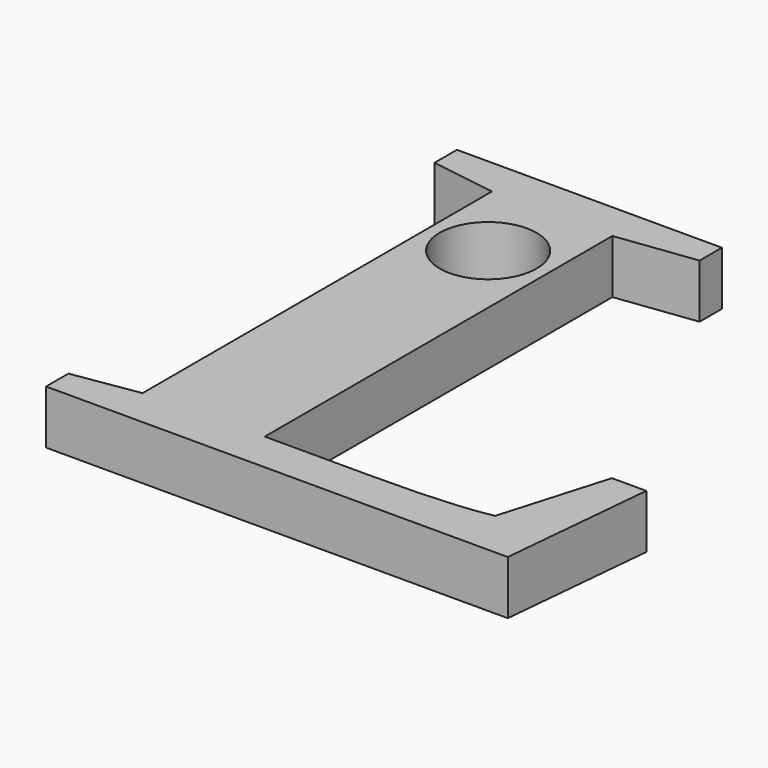
from build123d import *

# Parameters (mm, degrees)
F0_TEXT_SIZE = 72.7272727273
F1_DEPTH     = 5
F3_D         = 9


# Not quite as in the source:
# - Text() gives the source's letters only with a copy of the font that has no kerning and outlines rounded to 1/6400 em; it was checked with that copy


with BuildPart() as f1:
    # F0 (on Top) → F1 (new body)
    with BuildSketch(Plane.XY):
        with Locations((-41.6577126533, -22.5778426675)):
            Text('L', F0_TEXT_SIZE, font='Tinos', font_style=FontStyle.BOLD, text_align=(TextAlign.LEFT, TextAlign.BOTTOM))
    extrude(amount=F1_DEPTH)

    # F3 (through all)
    with Locations(Plane.XY.offset(5)):
        with Locations((-28.7145308351, 14.091167599)):
            Hole(F3_D / 2)


solid = f1.part
